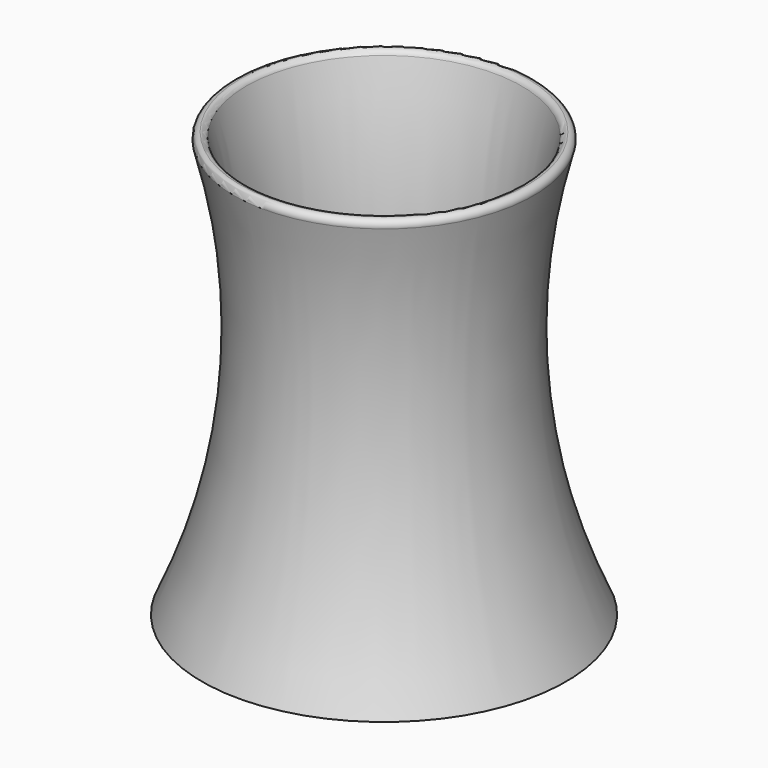
from build123d import *

# Parameters (mm, degrees)
F2_T = -50.8


# Not quite as in the source:
# - a fillet or chamfer that OpenCascade refuses, or shapes differently, is made with other operations: its cross-section is extruded or revolved along the edge and cut away or added


with BuildPart() as f1:
    # F0 (on Front) → F1 (revolve)
    with BuildSketch(Plane.XZ):
        with BuildLine():
            Line((-762, 0), (0, 0))
            Line((0, 0), (0, 1778))
            Line((0, 1778), (-635, 1778))
            ThreePointArc((-635, 1778), (-537.4071698995, 877.4933692785), (-762, 0))
        make_face()
    revolve(axis=Axis((0, 0, 889), (0, 0, -1)))

    # F2
    f2_openings = [f1.faces().sort_by_distance(p)[0] for p in [
        (0, 0, 1778),
    ]]
    offset(amount=F2_T, openings=f2_openings)

    # F3: fillet of radius 25.4 on 2 edges, made by hand

    # F3_s1 → F3_t2 (revolve, cut)
    with BuildSketch(Plane.XZ):
        with BuildLine():
            ThreePointArc((-601.2462046198, 1778), (-585.9068056848, 1772.845069531), (-576.7936693441, 1759.4726645916))
            ThreePointArc((-576.7936693441, 1759.4726645916), (-579.4173103836, 1768.7412417508), (-582.075394382, 1778))
            Line((-582.075394382, 1778), (-601.2462046198, 1778))
        make_face()
    revolve(axis=Axis((0, 0, 1778), (0, 0, 1)), mode=Mode.SUBTRACT)

    # F3_s3 → F3_t4 (revolve, cut)
    with BuildSketch(Plane.XZ):
        with BuildLine():
            ThreePointArc((-625.6987398956, 1745.7273354084), (-621.4912741508, 1767.939398935), (-601.2462046198, 1778))
            Line((-601.2462046198, 1778), (-635, 1778))
            ThreePointArc((-635, 1778), (-630.296026904, 1761.8790416292), (-625.6987398956, 1745.7273354084))
        make_face()
    revolve(axis=Axis((0, 0, 1778), (0, 0, -1)), mode=Mode.SUBTRACT)


solid = f1.part
